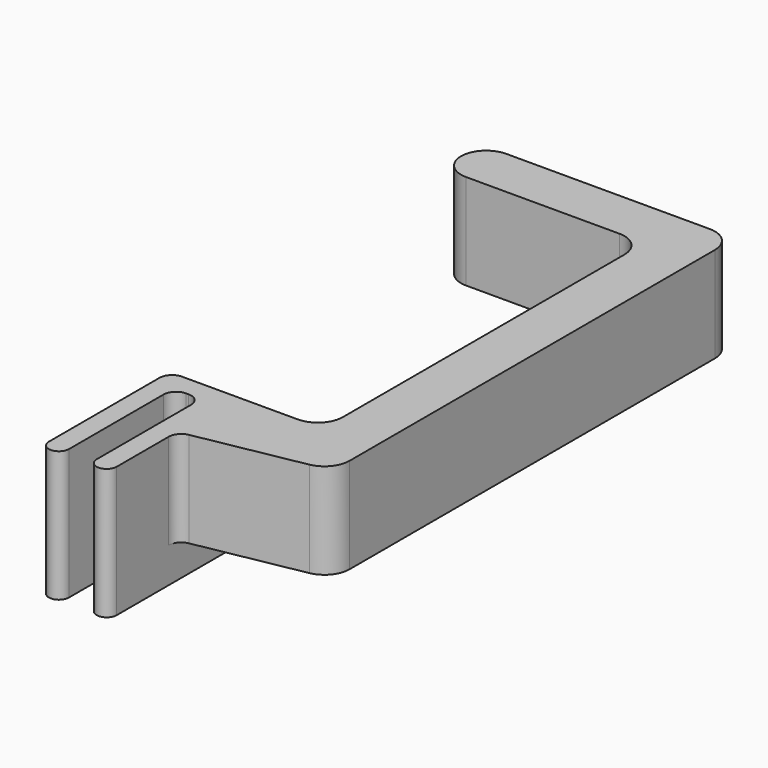
from build123d import *

# Parameters (mm, degrees)
F1_DEPTH = 26
F3_DEPTH = 7
F4_R     = 5
F5_R     = 2.5


with BuildPart() as f1:
    # F0 (on Top) → F1 (new body)
    with BuildSketch(Plane.XY):
        Polygon((0, 30), (0, 0), (4, 0), (4, 26), (9.5, 26), (9.5, 0), (13.5, 0), (13.5, 15), (40.5, 20), (40.5, 120), (30.5, 120), (-5, 120), (-5, 110), (30.5, 110), (30.5, 30), align=None)
        with BuildLine():
            Line((4, 0), (0, 0))
            ThreePointArc((0, 0), (2, -2), (4, 0))
        make_face()
        with BuildLine():
            ThreePointArc((-5, 120), (-10, 115), (-5, 110))
            Line((-5, 110), (-5, 120))
        make_face()
        with BuildLine():
            Line((13.5, 0), (9.5, 0))
            ThreePointArc((9.5, 0), (11.5, -2), (13.5, 0))
        make_face()
    extrude(amount=F1_DEPTH)

    # F2 (on face) → F3 (cut)
    with BuildSketch(Plane(origin=(0, 0, 0), x_dir=(1, 0, 0), z_dir=(0, 0, -1))):
        with BuildLine():
            Line((13.5, -30), (30.5, -30))
            Line((30.5, -30), (30.5, -110))
            Line((30.5, -110), (-5, -110))
            ThreePointArc((-5, -110), (-10, -115), (-5, -120))
            Line((-5, -120), (13.5, -120))
            Line((13.5, -120), (40.5, -120))
            Line((40.5, -120), (40.5, -20))
            Line((40.5, -20), (13.5, -15))
            Line((13.5, -15), (13.5, -30))
        make_face()
    extrude(amount=-F3_DEPTH, mode=Mode.SUBTRACT)

    # F4
    f4_edges = [f1.edges().sort_by_distance(p)[0] for p in [
        (40.5, 120, 16.5),
        (30.5, 110, 16.5),
        (30.5, 30, 16.5),
        (40.5, 20, 16.5),
    ]]
    fillet(f4_edges, radius=F4_R)

    # F5
    f5_edges = [f1.edges().sort_by_distance(p)[0] for p in [
        (0, 30, 13),
        (4, 26, 13),
        (9.5, 26, 13),
        (13.5, 15, 16.5),
        (13.5, 30, 3.5),
    ]]
    fillet(f5_edges, radius=F5_R)


solid = f1.part
